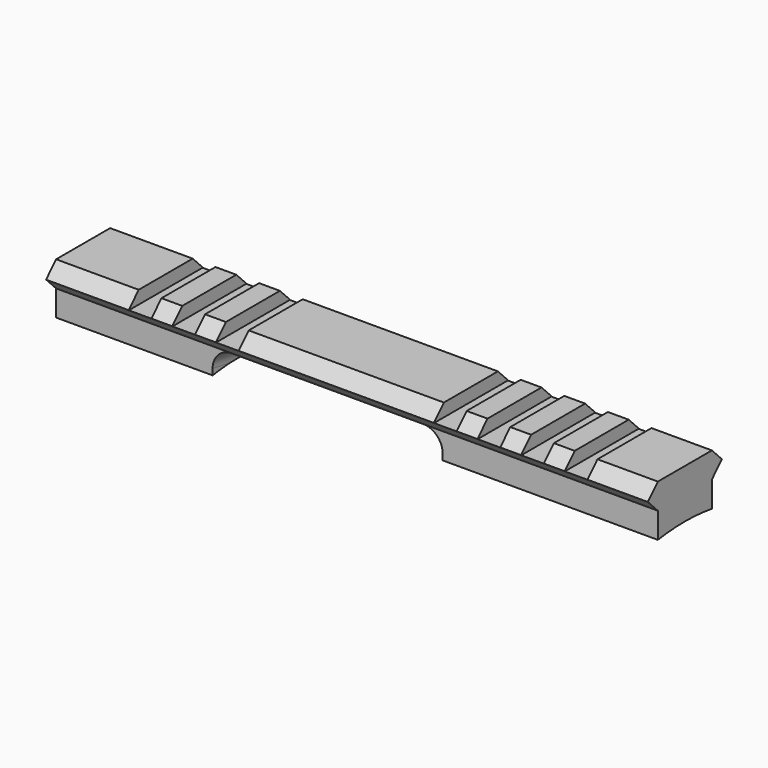
from build123d import *

# Parameters (mm, degrees)
F1_DEPTH  = 69.05625
F4_ANGLE  = 90
F5_W      = 5.2284544853
F5_H      = 7.121348225
F6_DEPTH  = 12.7
F7_W      = 52.8066
F7_H      = 18.3185085185
F7_H_2    = 5.8928
F9_DEPTH  = 25.4
F10_ANGLE = 350
F12_R     = 4.445
F14_DEPTH = 1.5875


# Not quite as in the source:
# - a feature names something its author has since deleted; it is built from what else it names


with BuildPart() as f1:
    # F0 (on Right) → F1 (new body, symmetric)
    with BuildSketch(Plane.YZ):
        with BuildLine():
            ThreePointArc((15.8326655208, 0), (15.688324924, -3.8842128409), (15.2560993298, -7.747))
            Line((15.2560993298, -7.747), (21.1488993298, -7.747))
            Line((21.1488993298, -7.747), (24.0952993298, -10.6299))
            Line((24.0952993298, -10.6299), (27.0416993298, -7.747))
            Line((27.0416993298, -7.747), (27.0416993298, 0))
            Line((27.0416993298, 0), (15.8326655208, 0))
        make_face()
    extrude(amount=F1_DEPTH, both=True)

    # F2: F1 across plane


with BuildPart() as f1_1:
    add(f1.part)
    add(f1.part.mirror(Plane.XY))


with BuildPart() as f1_2:
    # F4: moved
    add(f1_1.part.rotate(Axis((39.1787812114, 0, 0), (1, 0, 0)), F4_ANGLE))

    # F5 (on Front) → F6 (cut, symmetric)
    with BuildSketch(Plane.XZ):
        with Locations((-47.4936227574, 27.6051734423)):
            Rectangle(F5_W, F5_H)
        with Locations((-37.4860227574, 27.6051734423)):
            Rectangle(F5_W, F5_H)
        with Locations((-27.4784227574, 27.6051734423)):
            Rectangle(F5_W, F5_H)
        with Locations((22.5595772426, 27.6051734423)):
            Rectangle(F5_W, F5_H)
        with Locations((32.5671772426, 27.6051734423)):
            Rectangle(F5_W, F5_H)
        with Locations((42.5747772426, 27.6051734423)):
            Rectangle(F5_W, F5_H)
        with Locations((52.5823772426, 27.6051734423)):
            Rectangle(F5_W, F5_H)
    extrude(amount=F6_DEPTH, both=True, mode=Mode.SUBTRACT)


with BuildPart() as f9:
    # F7 (on face) → F9 (new body)
    with BuildSketch(Plane.XZ.offset(7.747)):
        with Locations((-6.73735, 6.0968450705)):
            Rectangle(F7_W, F7_H)
        with Locations((-6.73735, 18.2024993298)):
            Rectangle(F7_W, F7_H_2)
    extrude(amount=-F9_DEPTH)


with BuildPart() as f9_1:
    # F10: moved
    add(f9.part.rotate(Axis((-6.73735, -7.747, 21.1488993298), (1, 0, 0)), F10_ANGLE))


with BuildPart() as f1_3:
    add(f1_2.part)

    # F11: cut F9
    add(f9_1.part, mode=Mode.SUBTRACT)

    # F12
    f12_edges = [f1_3.edges().sort_by_distance(p)[0] for p in [
        (-33.14065, 0, 19.782894),
        (19.66595, 0, 19.782894),
    ]]
    fillet(f12_edges, radius=F12_R)

    # F13 (on face) → F14 (join)
    with BuildSketch(Plane(origin=(19.66595, 0, 0), x_dir=(0, -1, 0), z_dir=(-1, 0, 0))):
        Polygon((-7.7439094894, 15.2560993298), (7.747, 15.2560993298), (7.747, 16.6353280399), (-7.7439094894, 16.5785290301), align=None)
    extrude(amount=-F14_DEPTH)


solid = f1_3.part
